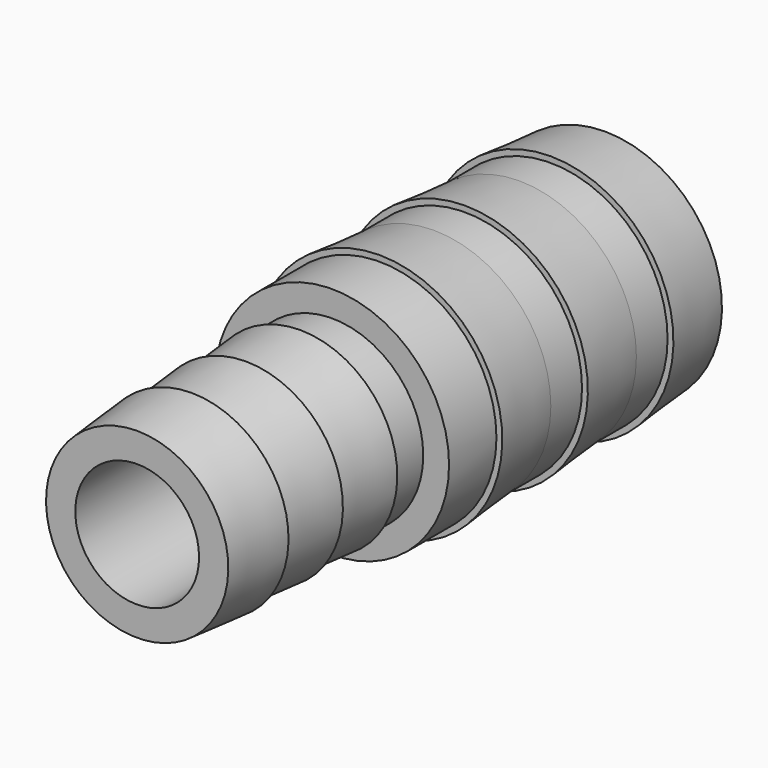
from build123d import *

# Parameters (mm, degrees)
F0_R          = 4.675
F0_R_2        = 3.175
F1_DEPTH      = 15
F1_DEPTH_BACK = 2.5
F2_R          = 6
F2_R_2        = 4.5
F3_DEPTH      = 15
F3_DEPTH_BACK = 2.5


# Not quite as in the source:
# - a fillet or chamfer that OpenCascade refuses, or shapes differently, is made with other operations: its cross-section is extruded or revolved along the edge and cut away or added


with BuildPart() as f1:
    # F0 (on Front) → F1 (new body, two sides)
    with BuildSketch(Plane.XZ) as f1_sk:
        Circle(F0_R)
        Circle(F0_R_2, mode=Mode.SUBTRACT)
    extrude(amount=F1_DEPTH)
    extrude(f1_sk.sketch, amount=-F1_DEPTH_BACK)

    # F2 (on Front) → F3 (join, two sides)
    with BuildSketch(Plane.XZ) as f3_sk:
        Circle(F2_R)
        Circle(F2_R_2, mode=Mode.SUBTRACT)
    extrude(amount=-F3_DEPTH)
    extrude(f3_sk.sketch, amount=F3_DEPTH_BACK)

    # F4 (on Right) → F5 (revolve)
    with BuildSketch(Plane.YZ):
        Polygon((-4.5386425355, 4.975), (-8.0257616903, 4.675), (-4.5386425355, 4.675), align=None)
        Polygon((-8.0257616903, 4.975), (-11.5128808452, 4.675), (-8.0257616903, 4.675), align=None)
        Polygon((-11.5128808452, 4.975), (-15, 4.675), (-11.5128808452, 4.675), align=None)
        Polygon((11.5128808452, 6), (15, 6), (11.5128808452, 6.3), align=None)
        Polygon((6.0257616903, 6), (9.5128808452, 6), (6.0257616903, 6.3), align=None)
        Polygon((0.5386425355, 6), (4.0257616903, 6), (0.5386425355, 6.3), align=None)
    revolve(axis=Axis((0, -13.8101289049, 0), (0, -1, 0)))

    # F6: fillet of radius 5 on 1 edges, made by hand

    # F6_s1 → F6_t2 (revolve, cut)
    with BuildSketch(Plane.XY):
        with BuildLine():
            ThreePointArc((3.175, -0.8903355291), (3.5180159975, 0.9296919432), (4.5, 2.5))
            Line((4.5, 2.5), (4.4265, 2.5678067106))
            ThreePointArc((4.4265, 2.5678067106), (3.8375, 2.6), (3.175, 2.6))
            Line((3.175, 2.6), (3.075, 2.5))
            Line((3.075, 2.5), (3.075, -0.8903355291))
            Line((3.075, -0.8903355291), (3.175, -0.8903355291))
        make_face()
    revolve(axis=Axis((0, 2.5, 0), (0, -1, 0)), mode=Mode.SUBTRACT)


solid = f1.part
